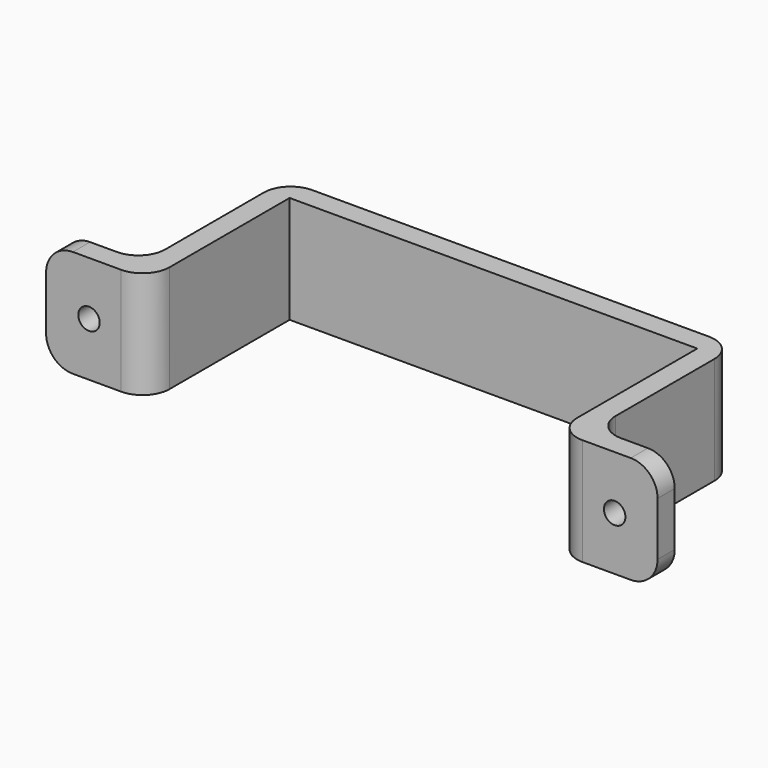
from build123d import *

# Parameters (mm, degrees)
F1_DEPTH = 20
F2_R     = 2
F3_DEPTH = 25
F4_R     = 4.99999


# Not quite as in the source:
# - a fillet or chamfer is up to 0.001 mm smaller than in the source, because OpenCascade refuses the exact size


with BuildPart() as f1:
    # F0 (on Top) → F1 (new body)
    with BuildSketch(Plane.XY):
        Polygon((-38, 33), (0, 33), (0, 37), (-42, 37), (-42, 4), (-57, 4), (-57, 0), (-38, 0), align=None)
        Polygon((0, 37), (0, 33), (38, 33), (38, 0), (57, 0), (57, 4), (42, 4), (42, 37), align=None)
    extrude(amount=F1_DEPTH)

    # F2 (on face) → F3 (cut)
    with BuildSketch(Plane(origin=(0, 4, 0), x_dir=(-1, 0, 0), z_dir=(0, 1, 0))):
        with Locations((49, 10)):
            Circle(F2_R)
        with Locations((-49, 10)):
            Circle(F2_R)
    extrude(amount=-F3_DEPTH, mode=Mode.SUBTRACT)

    # F4 (radius 5 in the source; OpenCascade refuses exactly that, so slightly less here)
    f4_edges = [f1.edges().sort_by_distance(p)[0] for p in [
        (-57, 2, 20),
        (-57, 2, 0),
        (57, 2, 0),
        (57, 2, 20),
        (42, 37, 10),
        (-42, 37, 10),
        (-38, 0, 10),
        (38, 0, 10),
        (42, 4, 10),
        (-42, 4, 10),
    ]]
    fillet(f4_edges, radius=F4_R)


solid = f1.part
